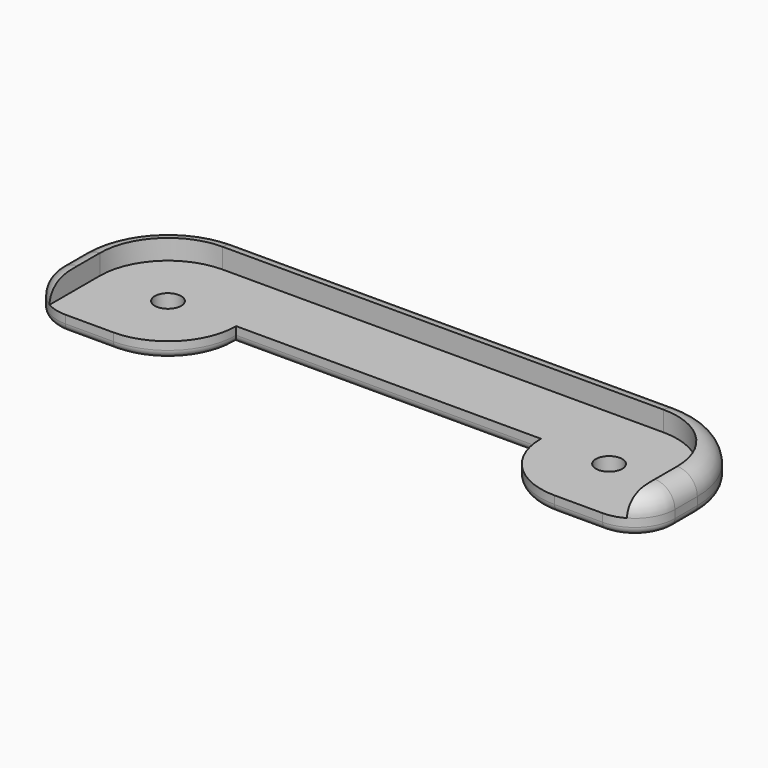
from build123d import *

# Parameters (mm, degrees)
F1_DEPTH = 2.5
F2_DEPTH = 2
F3_D     = 3.3
F4_R     = 5
F5_R     = 2.49999
F6_R     = 1


# Not quite as in the source:
# - a fillet or chamfer is up to 0.001 mm smaller than in the source, because OpenCascade refuses the exact size


with BuildPart() as f1:
    # F0 (on Top) → F1 (new body)
    with BuildSketch(Plane.XY):
        with BuildLine():
            ThreePointArc((-36, 0), (-33.5104076401, 6.0104076401), (-27.5, 8.5))
            Line((-27.5, 8.5), (27.5, 8.5))
            ThreePointArc((27.5, 8.5), (33.5104076401, 6.0104076401), (36, 0))
            Line((36, 0), (36, -8.5))
            Line((36, -8.5), (38.4999999404, -8.5))
            Line((38.4999999404, -8.5), (38.4999999404, 0))
            ThreePointArc((38.4999999404, 0), (35.2781745509, 7.7781745509), (27.5, 10.9999999404))
            Line((27.5, 10.9999999404), (-27.5, 10.9999999404))
            ThreePointArc((-27.5, 10.9999999404), (-35.2781745509, 7.7781745509), (-38.4999999404, 0))
            Line((-38.4999999404, 0), (-38.4999999404, -8.5))
            Line((-38.4999999404, -8.5), (-36, -8.5))
            Line((-36, -8.5), (-36, 0))
        make_face()
    extrude(amount=F1_DEPTH)

    # F0 (on Top) → F2 (join)
    with BuildSketch(Plane.XY):
        with BuildLine():
            ThreePointArc((-36, 0), (-33.5104076401, 6.0104076401), (-27.5, 8.5))
            Line((-27.5, 8.5), (27.5, 8.5))
            ThreePointArc((27.5, 8.5), (33.5104076401, 6.0104076401), (36, 0))
            Line((36, 0), (36, -8.5))
            Line((36, -8.5), (38.4999999404, -8.5))
            Line((38.4999999404, -8.5), (38.4999999404, 0))
            ThreePointArc((38.4999999404, 0), (35.2781745509, 7.7781745509), (27.5, 10.9999999404))
            Line((27.5, 10.9999999404), (-27.5, 10.9999999404))
            ThreePointArc((-27.5, 10.9999999404), (-35.2781745509, 7.7781745509), (-38.4999999404, 0))
            Line((-38.4999999404, 0), (-38.4999999404, -8.5))
            Line((-38.4999999404, -8.5), (-36, -8.5))
            Line((-36, -8.5), (-36, 0))
        make_face()
        with BuildLine():
            Line((27.5, 8.5), (-27.5, 8.5))
            ThreePointArc((-27.5, 8.5), (-33.5104076401, 6.0104076401), (-36, 0))
            Line((-36, 0), (-36, -8.5))
            Line((-36, -8.5), (-27.5, -8.5))
            ThreePointArc((-27.5, -8.5), (-21.4895923599, -6.0104076401), (-19, 0))
            Line((-19, 0), (19, 0))
            ThreePointArc((19, 0), (21.4895923599, -6.0104076401), (27.5, -8.5))
            Line((27.5, -8.5), (36, -8.5))
            Line((36, -8.5), (36, 0))
            ThreePointArc((36, 0), (33.5104076401, 6.0104076401), (27.5, 8.5))
        make_face()
    extrude(amount=-F2_DEPTH)

    # F3 (through all)
    with Locations(Plane.XY):
        with Locations((27.5, 0), (-27.5, 0)):
            Hole(F3_D / 2)

    # F4
    f4_edges = [f1.edges().sort_by_distance(p)[0] for p in [
        (-38.5, -8.5, 0.25),
        (38.5, -8.5, 0.25),
    ]]
    fillet(f4_edges, radius=F4_R)

    # F5 (radius 2.5 in the source; OpenCascade refuses exactly that, so slightly less here)
    f5_edges = [f1.edges().sort_by_distance(p)[0] for p in [
        (0, 11, 2.5),
    ]]
    fillet(f5_edges, radius=F5_R)

    # F6
    f6_edges = [f1.edges().sort_by_distance(p)[0] for p in [
        (0, 11, -2),
        (0, 0, -2),
    ]]
    fillet(f6_edges, radius=F6_R)


solid = f1.part
